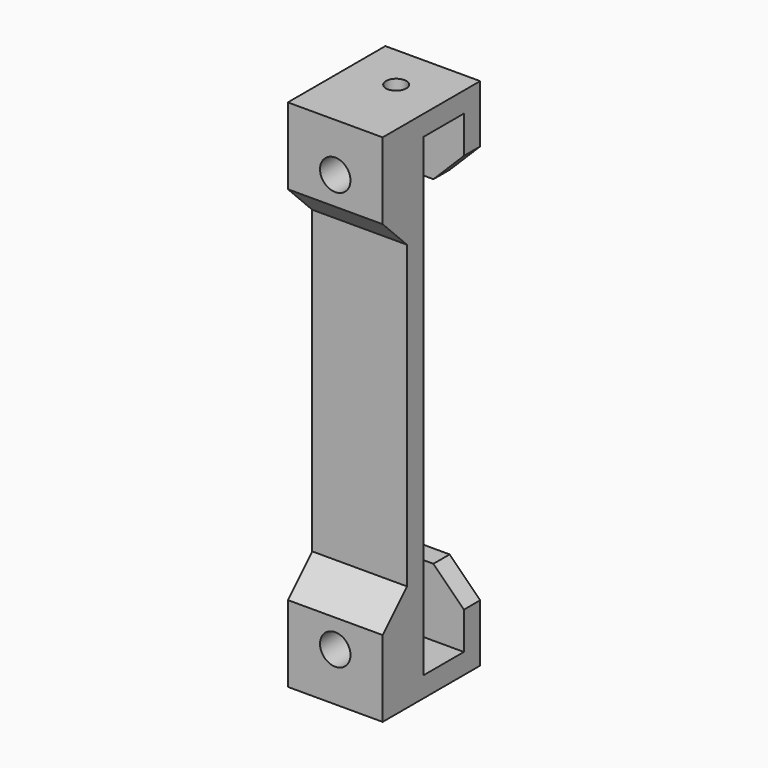
from build123d import *

# Parameters (mm, degrees)
F1_DEPTH = 7
F2_SIZE  = 4.49999
F3_R     = 2.25
F4_DEPTH = 7.5
F5_R     = 1.5
F6_DEPTH = 76.001


# Not quite as in the source:
# - a fillet or chamfer is up to 0.001 mm smaller than in the source, because OpenCascade refuses the exact size


with BuildPart() as f1:
    # F0 (on Right) → F1 (new body, symmetric)
    with BuildSketch(Plane.YZ):
        Polygon((-3.75, 35), (3.75, 35), (3.75, 25), (6.75, 25), (6.75, 38), (-11.25, 38), (-11.25, 26.71), (-6.75, 26.71), (-6.75, -26.71), (-11.25, -26.71), (-11.25, -38), (6.75, -38), (6.75, -25), (3.75, -25), (3.75, -35), (-3.75, -35), align=None)
    extrude(amount=F1_DEPTH, both=True)

    # F2 (size 4.5 in the source; OpenCascade refuses exactly that, so slightly less here)
    f2_edges = [f1.edges().sort_by_distance(p)[0] for p in [
        (0, -6.75, 26.71),
        (0, -6.75, -26.71),
        (-7, 5.25, 25),
        (7, 5.25, 25),
        (-7, 5.25, -25),
        (7, 5.25, -25),
    ]]
    chamfer(f2_edges, length=F2_SIZE)

    # F3 (on face) → F4 (cut, through all)
    with BuildSketch(Plane.XZ.offset(11.25)):
        with Locations((0, 30.855)):
            Circle(F3_R)
        with Locations((0, -30.855)):
            Circle(F3_R)
    extrude(amount=-F4_DEPTH, mode=Mode.SUBTRACT)

    # F5 (on face) → F6 (cut, through all)
    with BuildSketch(Plane.XY.offset(38)):
        Circle(F5_R)
    extrude(amount=-F6_DEPTH, mode=Mode.SUBTRACT)


solid = f1.part
